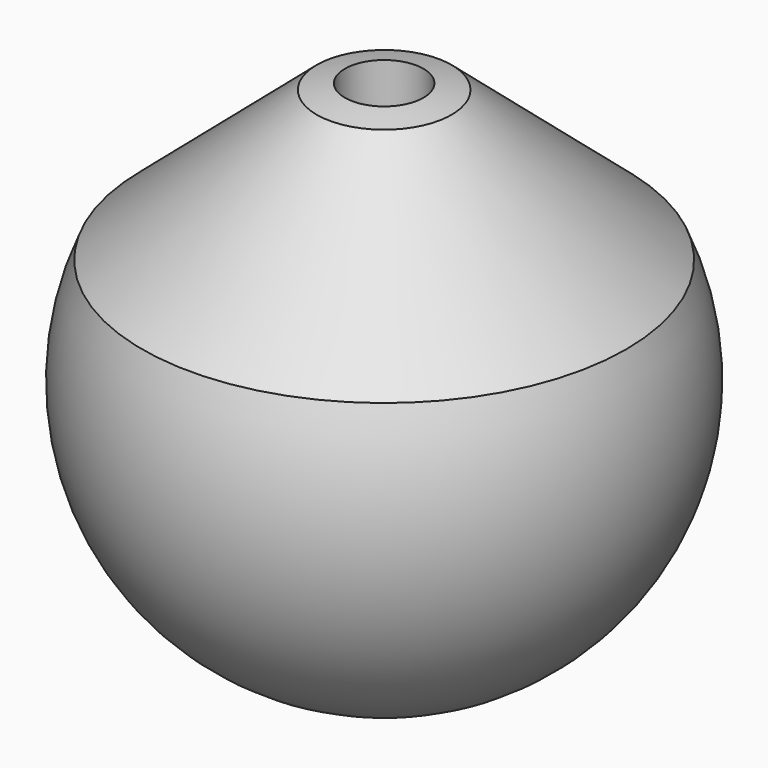
from build123d import *

# Parameters (mm, degrees)
F0_W = 4.7244
F0_H = 9.525


# Not quite as in the source:
# - a feature names something its author has since deleted; it is built from what else it names


with BuildPart() as f1:
    # F0 (on Front) → F1 (revolve)
    with BuildSketch(Plane.XZ):
        with BuildLine():
            Line((-8.1087104998, 34.5070896671), (-22.5402639736, 16.51))
            ThreePointArc((-22.5402639736, 16.51), (-25.8838273037, -10.5200325148), (-4.6314331906, -27.5534648747))
            Line((-4.6314331906, -27.5534648747), (-1.6002, -27.8064487898))
            Line((-1.6002, -27.8064487898), (-1.6002, -5.842))
            Line((-1.6002, -5.842), (0, -5.842))
            Line((0, -5.842), (0, 0))
            Line((0, 0), (0, 3.81))
            Line((0, 3.81), (0, 16.51))
            Line((0, 16.51), (-4.7244, 16.51))
            Line((-4.7244, 16.51), (-4.7244, 26.035))
            Line((-4.7244, 26.035), (-4.7244, 35.2065371441))
            ThreePointArc((-4.7244, 35.2065371441), (-6.4260787397, 34.9028932721), (-8.1087104998, 34.5070896671))
        make_face()
        with Locations((-2.3622, 21.2725)):
            Rectangle(F0_W, F0_H)
        with BuildLine():
            Line((0, 0), (0, -5.842))
            Line((0, -5.842), (0, -25.4))
            ThreePointArc((0, -25.4), (23.0706956982, -10.625582337), (19.302328875, 16.51))
            Line((19.302328875, 16.51), (0, 16.51))
            Line((0, 16.51), (0, 3.81))
            Line((0, 3.81), (0, 0))
        make_face()
    revolve(axis=Axis((0, 0, 3.81), (0, 0, 1)))

    # F0 (on Front) → F2 (revolve)
    with BuildSketch(Plane.XZ):
        with BuildLine():
            Line((-8.1087104998, 34.5070896671), (-22.5402639736, 16.51))
            ThreePointArc((-22.5402639736, 16.51), (-25.8838273037, -10.5200325148), (-4.6314331906, -27.5534648747))
            Line((-4.6314331906, -27.5534648747), (-1.6002, -27.8064487898))
            Line((-1.6002, -27.8064487898), (-1.6002, -5.842))
            Line((-1.6002, -5.842), (0, -5.842))
            Line((0, -5.842), (0, 0))
            Line((0, 0), (0, 3.81))
            Line((0, 3.81), (0, 16.51))
            Line((0, 16.51), (-4.7244, 16.51))
            Line((-4.7244, 16.51), (-4.7244, 26.035))
            Line((-4.7244, 26.035), (-4.7244, 35.2065371441))
            ThreePointArc((-4.7244, 35.2065371441), (-6.4260787397, 34.9028932721), (-8.1087104998, 34.5070896671))
        make_face()
        with BuildLine():
            ThreePointArc((-4.6314331906, -27.5534648747), (-25.8838273037, -10.5200325148), (-22.5402639736, 16.51))
            Line((-22.5402639736, 16.51), (-29.099355663, 16.51))
            ThreePointArc((-29.099355663, 16.51), (-27.9182626522, -11.3106187202), (-5.2629922621, -27.5007555394))
            Line((-5.2629922621, -27.5007555394), (-4.6314331906, -27.5534648747))
        make_face()
        Polygon((-29.099355663, 16.51), (-22.5402639736, 16.51), (-8.1087104998, 34.5070896671), align=None)
    revolve(axis=Axis((0, 0, -12.065), (0, 0, 1)))


solid = f1.part
